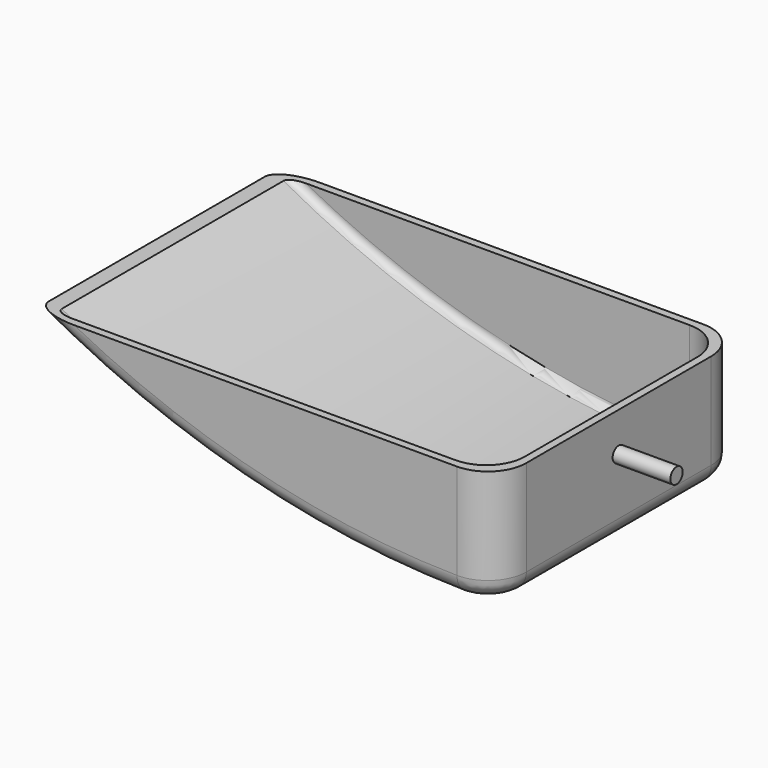
from build123d import *

# Parameters (mm, degrees)
F2_DEPTH     = 101.6
F3_T         = -5.08
F0_R         = 5.08
F4_DEPTH     = 38.1
F5_T4_DEPTH  = 134.2759536589
F5_S5_R      = 576.6246219757
F5_T6_DEPTH  = 71
F5_T10_DEPTH = 134.2759536589
F5_S11_R     = 576.6246219757
F5_T12_DEPTH = 71
F5_T13_DEPTH = 202.727744005
F6_R         = 12.7
F7_R         = 5.08


# Not quite as in the source:
# - a fillet or chamfer that OpenCascade refuses, or shapes differently, is made with other operations: its cross-section is extruded or revolved along the edge and cut away or added


with BuildPart() as f2:
    # F1 (on Front) → F2 (new body, symmetric)
    with BuildSketch(Plane.XZ):
        with BuildLine():
            Line((0, -49.880515784), (0, 25.847228221))
            Line((0, 25.847228221), (-304.8, 25.847228221))
            ThreePointArc((-304.8, 25.847228221), (-157.6074099904, -32.9761822695), (0, -49.880515784))
        make_face()
    extrude(amount=F2_DEPTH, both=True)

    # F3
    f3_openings = [f2.faces().sort_by_distance(p)[0] for p in [
        (-152.4, 0, 25.847228),
    ]]
    offset(amount=F3_T, openings=f3_openings)

    # F0 (on Right) → F4 (join)
    with BuildSketch(Plane.YZ):
        Circle(F0_R)
    extrude(amount=F4_DEPTH)

    # F5: fillet of radius 25.4 on 4 edges, made by hand


with BuildPart() as f5_tool2:
    # F5_s3 → F5_t4 (new body)
    with BuildSketch(Plane.XY.offset(25.847228221)):
        with BuildLine():
            ThreePointArc((-5.08, -71.12), (-12.5194877579, -89.0805122421), (-30.48, -96.52))
            Line((-30.48, -96.52), (-5.08, -96.52))
            Line((-5.08, -96.52), (-5.08, -71.12))
        make_face()
    extrude(amount=-F5_T4_DEPTH)

    # F5_s5 → F5_t6 (intersect, symmetric)
    with BuildSketch(Plane.XZ.offset(83.8)):
        with Locations((-17.3467118203, 531.5654050176)):
            Circle(F5_S5_R)
    extrude(amount=F5_T6_DEPTH, both=True, mode=Mode.INTERSECT)


with BuildPart() as f2_1:
    add(f2.part)

    # F5_t1: union F5_tool2
    add(f5_tool2.part)


with BuildPart() as f5_tool8:
    # F5_s9 → F5_t10 (new body)
    with BuildSketch(Plane.XY.offset(25.847228221)):
        with BuildLine():
            ThreePointArc((-30.48, 96.52), (-12.5194877579, 89.0805122421), (-5.08, 71.12))
            Line((-5.08, 71.12), (-5.08, 96.52))
            Line((-5.08, 96.52), (-30.48, 96.52))
        make_face()
    extrude(amount=-F5_T10_DEPTH)

    # F5_s11 → F5_t12 (intersect, symmetric)
    with BuildSketch(Plane.XZ.offset(-83.8)):
        with Locations((-17.3467118203, 531.5654050176)):
            Circle(F5_S11_R)
    extrude(amount=F5_T12_DEPTH, both=True, mode=Mode.INTERSECT)


with BuildPart() as f2_2:
    add(f2_1.part)

    # F5_t7: union F5_tool8
    add(f5_tool8.part)

    # F5_s14 → F5_t13 (cut)
    with BuildSketch(Plane.XY.offset(-113.380515784)):
        with BuildLine():
            ThreePointArc((0, -76.2), (-7.4394877579, -94.1605122421), (-25.4, -101.6))
            Line((-25.4, -101.6), (0, -101.6))
            Line((0, -101.6), (0, -76.2))
        make_face()
        with BuildLine():
            ThreePointArc((0, 76.2), (-7.4394877579, 94.1605122421), (-25.4, 101.6))
            Line((-25.4, 101.6), (0, 101.6))
            Line((0, 101.6), (0, 76.2))
        make_face()
    extrude(amount=F5_T13_DEPTH, mode=Mode.SUBTRACT)

    # F6
    f6_edges = [f2_2.edges().sort_by_distance(p)[0] for p in [
        (-7.439388, -94.160412, -50.054842),
        (0, 0, -49.880516),
        (-169.899659, -101.6, -29.779289),
        (-5.918318, 92.497978, -50.026943),
        (-169.899659, 101.6, -29.779289),
    ]]
    fillet(f6_edges, radius=F6_R)

    # F7
    f7_edges = [f2_2.edges().sort_by_distance(p)[0] for p in [
        (-166.679144, -96.52, -25.386819),
        (-10.998525, -87.418225, -45.024272),
        (-5.08, 0, -44.928725),
        (-11.01893, 87.442584, -45.024496),
        (-166.679144, 96.52, -25.386819),
    ]]
    fillet(f7_edges, radius=F7_R)


solid = f2_2.part
